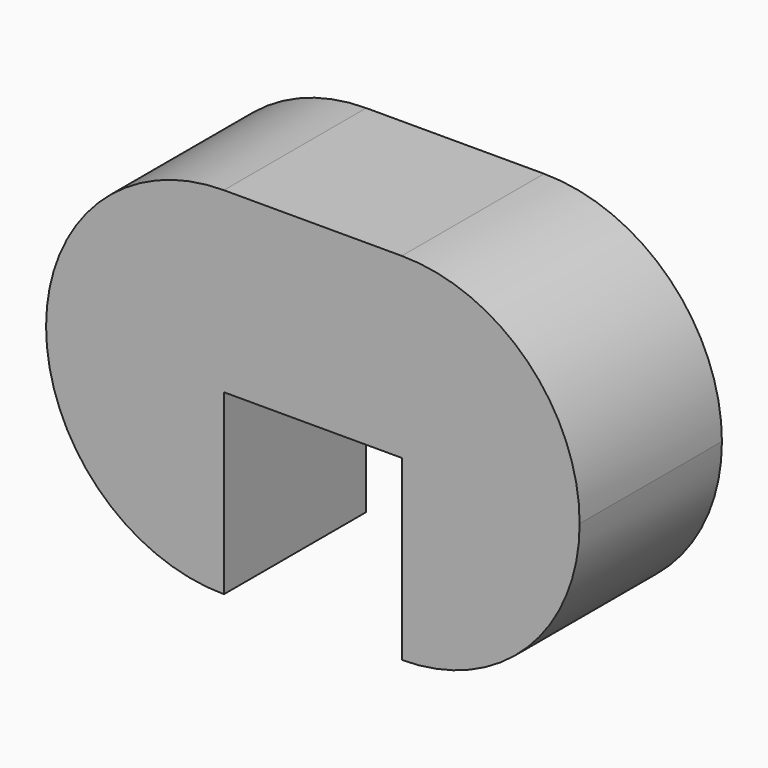
from build123d import *

# Parameters (mm, degrees)
F1_DEPTH = 5
F2_R     = 4.99999


# Not quite as in the source:
# - a fillet or chamfer is up to 0.001 mm smaller than in the source, because OpenCascade refuses the exact size


with BuildPart() as f1:
    # F0 (on Front) → F1 (new body)
    with BuildSketch(Plane.XZ):
        Polygon((-5, 0), (0, 0), (0, 5), (5, 5), (5, 0), (10, 0), (10, 10), (-5, 10), align=None)
    extrude(amount=F1_DEPTH)

    # F2 (radius 5 in the source; OpenCascade refuses exactly that, so slightly less here)
    f2_edges = [f1.edges().sort_by_distance(p)[0] for p in [
        (10, -2.5, 10),
        (10, -2.5, 0),
        (-5, -2.5, 10),
        (-5, -2.5, 0),
    ]]
    fillet(f2_edges, radius=F2_R)


solid = f1.part
